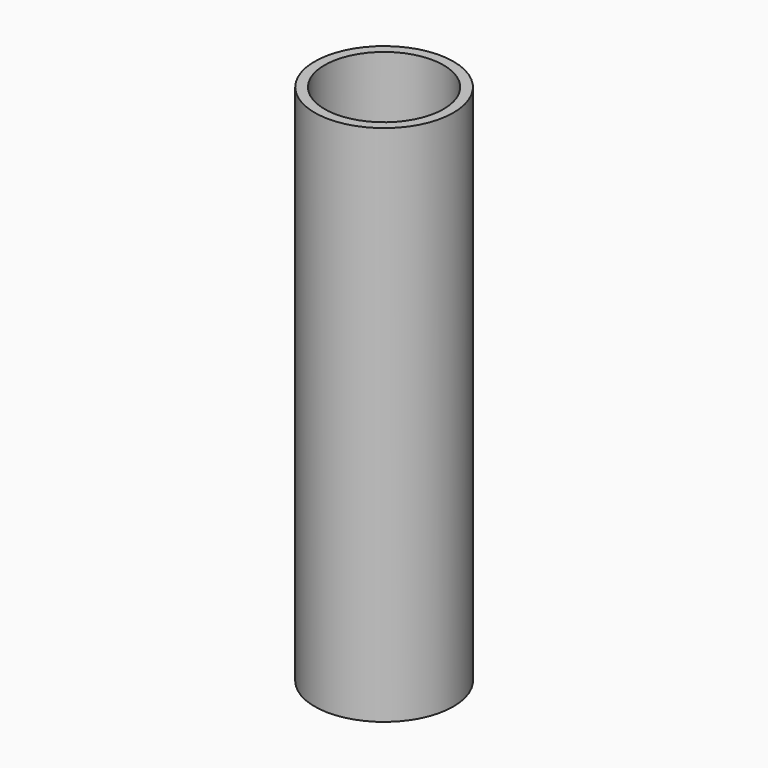
from build123d import *

# Parameters (mm, degrees)
F0_R     = 9.2921995523
F0_R_2   = 7.9676455341
F1_DEPTH = 70


# Not quite as in the source:
# - the program builds the solid bodies; features that only make, move or delete a surface that nothing else refers to are left out


with BuildPart() as f1:
    # F0 (on Top) → F1 (new body)
    with BuildSketch(Plane.XY):
        Circle(F0_R)
        Circle(F0_R_2, mode=Mode.SUBTRACT)
    extrude(amount=F1_DEPTH)


solid = f1.part
